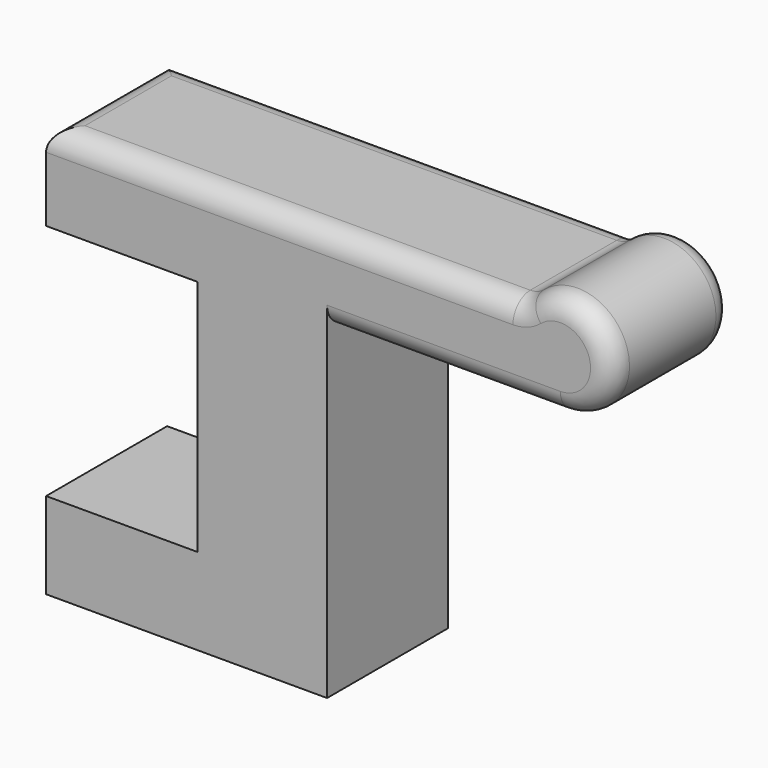
from build123d import *

# Parameters (mm, degrees)
F1_DEPTH = 35
F2_F1_R  = 5
F2_F2_R  = 5


with BuildPart() as f1:
    # F0 (on Front) → F1 (new body)
    with BuildSketch(Plane.XZ):
        with BuildLine():
            Line((0, 20), (0, 0))
            Line((0, 0), (65, 0))
            Line((65, 0), (65, 75))
            Line((65, 75), (118.94427191, 75))
            ThreePointArc((118.94427191, 75), (129.8987230601, 91.8989794856), (110, 95))
            Line((110, 95), (0, 95))
            Line((0, 95), (0, 75))
            Line((0, 75), (35, 75))
            Line((35, 75), (35, 20))
            Line((35, 20), (0, 20))
        make_face()
    extrude(amount=F1_DEPTH)

    # F2: fillet of radius 5 on 4 edges, made by hand

    # F2_f1
    f2_f1_edges = [f1.edges().sort_by_distance(p)[0] for p in [
        (110, -17.5, 95),
    ]]
    fillet(f2_f1_edges, radius=F2_F1_R)

    # F2_f2
    f2_f2_edges = [f1.edges().sort_by_distance(p)[0] for p in [
        (0, -17.5, 95),
        (53.9949103799, 0, 95),
        (53.9949103799, -35, 95),
        (109.7048066113, -35, 95.3033178169),
        (109.7048066113, 0, 95.3033178169),
    ]]
    fillet(f2_f2_edges, radius=F2_F2_R)


solid = f1.part
